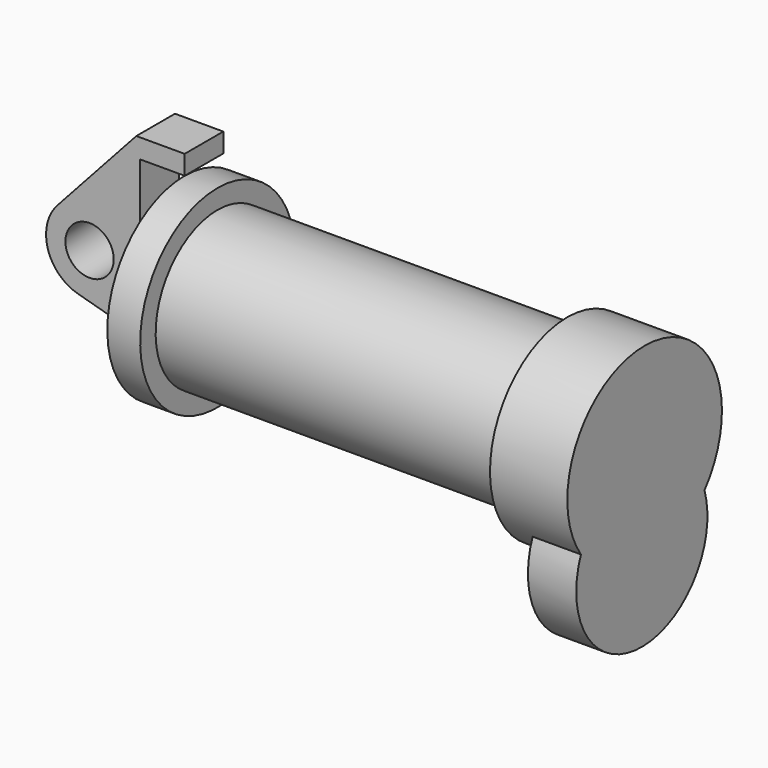
from build123d import *

# Parameters (mm, degrees)
F0_R     = 3.175
F1_DEPTH = 6.35
F5_DEPTH = 6.35


# Not quite as in the source:
# - a feature of the source that left no trace in its solid (it failed there, or was rolled back) is left out


with BuildPart() as f1:
    # F0 (on Front) → F1 (new body)
    with BuildSketch(Plane.XZ):
        with BuildLine():
            Line((-0.9398, 0), (0, 0))
            Line((0, 0), (0, 12.7))
            Line((0, 12.7), (5.842, 12.7))
            Line((5.842, 12.7), (5.842, 15.24))
            Line((5.842, 15.24), (-0.508, 15.24))
            Line((-0.508, 15.24), (-10.8806298187, 3.8475430269))
            ThreePointArc((-10.8806298187, 3.8475430269), (-4.5919612295, 5.3297205562), (-0.9398, 0))
        make_face()
        with BuildLine():
            ThreePointArc((-8.1826630726, -5.5069827884), (-3.1957909266, -4.5493385486), (-0.9398, 0))
            ThreePointArc((-0.9398, 0), (-4.5919612295, 5.3297205562), (-10.8806298187, 3.8475430269))
            ThreePointArc((-10.8806298187, 3.8475430269), (-12.1459778134, -1.5837270034), (-8.1826630726, -5.5069827884))
        make_face()
        with Locations((-6.6548, 0)):
            Circle(F0_R, mode=Mode.SUBTRACT)
        with BuildLine():
            Line((5.842, 0), (0, 0))
            Line((0, 0), (-0.9398, 0))
            ThreePointArc((-0.9398, 0), (-3.1957909266, -4.5493385486), (-8.1826630726, -5.5069827884))
            Line((-8.1826630726, -5.5069827884), (5.842, -9.398))
            Line((5.842, -9.398), (5.842, 0))
        make_face()
    extrude(amount=-F1_DEPTH)


with BuildPart() as f3:
    # F0 (on Front) → F3 (revolve)
    with BuildSketch(Plane.XZ):
        Polygon((5.842, 12.7), (5.842, 0), (66.294, 0), (66.294, 12.7), (56.134, 12.7), (56.134, 10.16), (10.16, 10.16), (10.16, 12.7), align=None)
    revolve(axis=Axis((33.147, 0, 0), (-1, 0, 0)))

    # F4 (on face) → F5 (join)
    with BuildSketch(Plane.YZ.offset(66.294)):
        with BuildLine():
            ThreePointArc((9.8396858807, -8.0293574942), (-0.5196744669, -12.6893632011), (-10.463295241, -7.1978783471))
            ThreePointArc((-10.463295241, -7.1978783471), (-0.8993069074, -21.9591931184), (9.8396858807, -8.0293574942))
        make_face()
        with BuildLine():
            Line((-9.8396858807, 8.0293574942), (-10.463295241, -7.1978783471))
            ThreePointArc((-10.463295241, -7.1978783471), (-0.5196744669, -12.6893632011), (9.8396858807, -8.0293574942))
            Line((9.8396858807, -8.0293574942), (10.463295241, 7.1978783471))
            Line((10.463295241, 7.1978783471), (-9.8396858807, 8.0293574942))
        make_face()
    extrude(amount=-F5_DEPTH)


solid = Compound([f1.part, f3.part])
